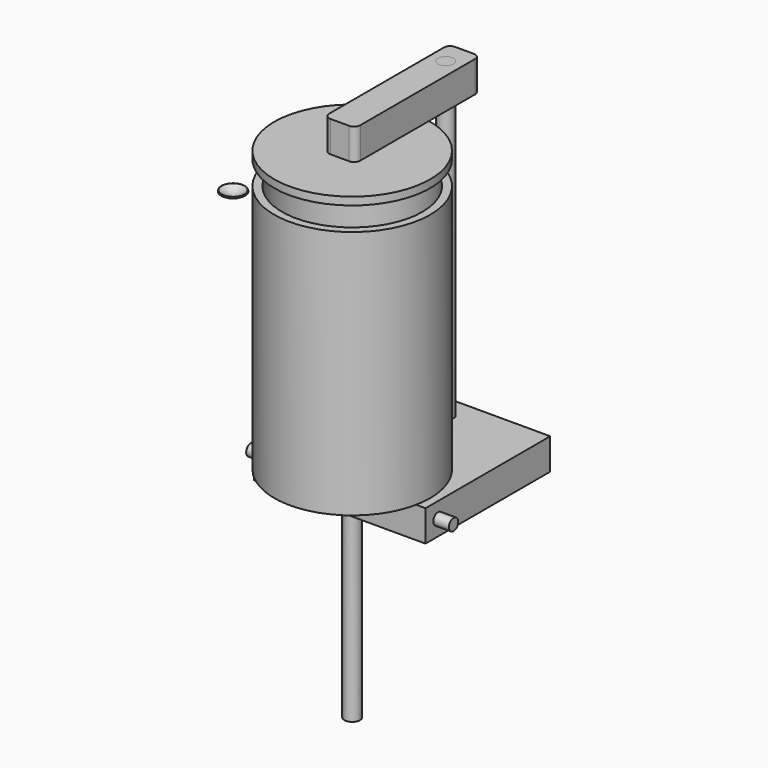
from build123d import *

# Parameters (mm, degrees)
F0_R      = 63.5
F1_DEPTH  = 203.2
F2_R      = 57.15
F3_DEPTH  = 190.5
F7_R      = 2.3876
F8_DEPTH  = 12.7
F9_W      = 139.7
F9_H      = 25.4
F9_R      = 2.54
F10_DEPTH = 25.4
F11_R     = 4.064
F12_DEPTH = 5.08
F14_R     = 6.35
F15_DEPTH = 152.4
F16_W     = 25.4
F16_H     = 127
F17_DEPTH = 25.4
F18_R     = 6.35
F19_DEPTH = 25.4
F20_R     = 6.35
F21_DEPTH = 304.8
F22_R     = 5.08
F23_W     = 139.7
F23_H     = 25.4
F24_DEPTH = 101.6
F25_R     = 6.35
F26_DEPTH = 279.401
F13_R     = 4.7625
F29_DEPTH = 12.7


with BuildPart() as f1:
    # F0 (on Top) → F1 (new body)
    with BuildSketch(Plane.XY):
        Circle(F0_R)
    extrude(amount=F1_DEPTH)

    # F2 (on face) → F3 (cut)
    with BuildSketch(Plane.XY.offset(203.2)):
        Circle(F2_R)
    extrude(amount=-F3_DEPTH, mode=Mode.SUBTRACT)

    # F7 (on face) → F8 (cut)
    with BuildSketch(Plane(origin=(0, 0, 0), x_dir=(1, 0, 0), z_dir=(0, 0, -1))):
        with Locations((-59.69, 0)):
            Circle(F7_R)
        with Locations((59.69, 0)):
            Circle(F7_R)
    extrude(amount=-F8_DEPTH, mode=Mode.SUBTRACT)


with BuildPart() as f6:
    # F5 (on Front) → F6 (revolve)
    with BuildSketch(Plane.XZ):
        Polygon((0, 215.9), (0, 228.6), (-63.5, 228.6), (-63.5, 222.25), (-54.1123329857, 222.25), (-50.8, 215.9), align=None)
    revolve(axis=Axis((0, 0, 222.25), (0, 0, 1)))


with BuildPart() as f10:
    # F9 (on face) → F10 (new body)
    with BuildSketch(Plane(origin=(0, 0, 0), x_dir=(1, 0, 0), z_dir=(0, 0, -1))):
        Rectangle(F9_W, F9_H)
        with Locations((-59.69, 0)):
            Circle(F9_R, mode=Mode.SUBTRACT)
        with Locations((59.69, 0)):
            Circle(F9_R, mode=Mode.SUBTRACT)
    extrude(amount=F10_DEPTH)

    # F11 (on face) → F12 (cut)
    with BuildSketch(Plane(origin=(0, 0, -25.4), x_dir=(1, 0, 0), z_dir=(0, 0, -1))):
        with Locations((-59.69, 0)):
            Circle(F11_R)
        with Locations((59.69, 0)):
            Circle(F11_R)
    extrude(amount=-F12_DEPTH, mode=Mode.SUBTRACT)

    # F23 (on face) → F24 (join)
    with BuildSketch(Plane(origin=(0, 12.7, 0), x_dir=(-1, 0, 0), z_dir=(0, 1, 0))):
        with Locations((0, -12.7)):
            Rectangle(F23_W, F23_H)
    extrude(amount=F24_DEPTH)

    # F25 (on face) → F26 (cut, through all)
    with BuildSketch(Plane(origin=(0, 0, -25.4), x_dir=(1, 0, 0), z_dir=(0, 0, -1))):
        with Locations((0, -95.25)):
            Circle(F25_R)
    extrude(amount=-F26_DEPTH, mode=Mode.SUBTRACT)


with BuildPart() as f15:
    # F14 (on face) → F15 (new body)
    with BuildSketch(Plane(origin=(0, 0, -25.4), x_dir=(1, 0, 0), z_dir=(0, 0, -1))):
        Circle(F14_R)
    extrude(amount=F15_DEPTH)


with BuildPart() as f17:
    # F16 (on face) → F17 (new body)
    with BuildSketch(Plane.XY.offset(228.6)):
        with Locations((0, 50.8)):
            Rectangle(F16_W, F16_H)
    extrude(amount=F17_DEPTH)

    # F18 (on face) → F19 (cut)
    with BuildSketch(Plane.XY.offset(254)):
        with Locations((0, 95.25)):
            Circle(F18_R)
    extrude(amount=-F19_DEPTH, mode=Mode.SUBTRACT)

    # F22
    f22_edges = [f17.edges().sort_by_distance(p)[0] for p in [
        (-12.7, -12.7, 241.3),
        (12.7, -12.7, 241.3),
        (12.7, 114.3, 241.3),
        (-12.7, 114.3, 241.3),
    ]]
    fillet(f22_edges, radius=F22_R)


with BuildPart() as f21:
    # F20 (on offset) → F21 (new body)
    with BuildSketch(Plane.XY.offset(254)):
        with Locations((0, 95.25)):
            Circle(F20_R)
    extrude(amount=-F21_DEPTH)


with BuildPart() as f28:
    # F27 (on Right) → F28 (revolve)
    with BuildSketch(Plane.YZ):
        with BuildLine():
            Line((-121.3002428412, 245.0738400221), (-121.3002428412, 246.0898400221))
            ThreePointArc((-121.3002428412, 246.0898400221), (-126.2048455265, 247.1539878791), (-130.5969267216, 249.5823949575))
            Line((-130.5969267216, 249.5823949575), (-130.7353358137, 249.5823949575))
            Line((-130.7353358137, 249.5823949575), (-131.0446783728, 248.6478379131))
            ThreePointArc((-131.0446783728, 248.6478379131), (-126.4637875903, 246.1662578068), (-121.3692276655, 245.0761847089))
            Line((-121.3692276655, 245.0761847089), (-121.3002428412, 245.0738400221))
        make_face()
    revolve(axis=Axis((0, -121.3002428412, 245.5818400221), (0, 0, -1)))


with BuildPart() as f29:
    # F13 (on face) → F29 (new body)
    with BuildSketch(Plane(origin=(-69.85, 0, 0), x_dir=(0, -1, 0), z_dir=(-1, 0, 0))):
        with Locations((0, -12.7)):
            Circle(F13_R)
    extrude(amount=F29_DEPTH)


with BuildPart() as f30_1:
    # F30: instance of F29
    add(f29.part.mirror(Plane.YZ))


solid = Compound([f1.part, f6.part, f10.part, f15.part, f17.part, f21.part, f28.part, f29.part, f30_1.part])
